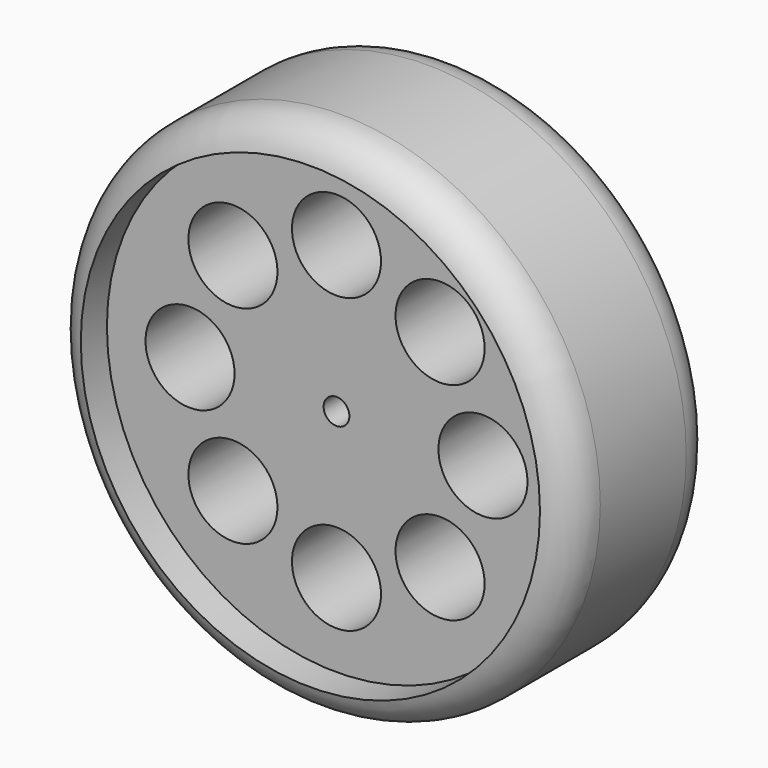
from build123d import *

# Parameters (mm, degrees)
F0_R     = 29.464
F0_R_2   = 5.715
F0_R_3   = 1.651
F1_DEPTH = 7.62
F0_R_4   = 33.274
F2_DEPTH = 11.811


# Not quite as in the source:
# - a fillet or chamfer that OpenCascade refuses, or shapes differently, is made with other operations: its cross-section is extruded or revolved along the edge and cut away or added


with BuildPart() as f1:
    # F0 (on Front) → F1 (new body, symmetric)
    with BuildSketch(Plane.XZ):
        Circle(F0_R)
        with Locations((-13.2907790592, -13.2907790592)):
            Circle(F0_R_2, mode=Mode.SUBTRACT)
        with Locations((0, -18.796)):
            Circle(F0_R_2, mode=Mode.SUBTRACT)
        with Locations((13.2907790592, -13.2907790592)):
            Circle(F0_R_2, mode=Mode.SUBTRACT)
        with Locations((-18.796, 0)):
            Circle(F0_R_2, mode=Mode.SUBTRACT)
        with Locations((-13.2907790592, 13.2907790592)):
            Circle(F0_R_2, mode=Mode.SUBTRACT)
        Circle(F0_R_3, mode=Mode.SUBTRACT)
        with Locations((13.2907790592, 13.2907790592)):
            Circle(F0_R_2, mode=Mode.SUBTRACT)
        with Locations((18.796, 0)):
            Circle(F0_R_2, mode=Mode.SUBTRACT)
        with Locations((0, 18.796)):
            Circle(F0_R_2, mode=Mode.SUBTRACT)
    extrude(amount=F1_DEPTH, both=True)

    # F0 (on Front) → F2 (join, symmetric)
    with BuildSketch(Plane.XZ):
        Circle(F0_R_4)
        Circle(F0_R, mode=Mode.SUBTRACT)
    extrude(amount=F2_DEPTH, both=True)

    # F3: fillet of radius 5.08 on 3 edges, made by hand

    # F3_s1 → F3_t2 (revolve, cut)
    with BuildSketch(Plane.XY):
        with BuildLine():
            ThreePointArc((33.274, 6.8923111503), (32.2100926284, 10.0031631237), (29.464, 11.811))
            Line((29.464, 11.811), (33.274, 11.811))
            Line((33.274, 11.811), (33.274, 6.8923111503))
        make_face()
    revolve(axis=Axis((0, 11.811, 0), (0, -1, 0)), mode=Mode.SUBTRACT)

    # F3_s3 → F3_t4 (revolve, cut)
    with BuildSketch(Plane.XY):
        with BuildLine():
            ThreePointArc((33.274, -6.8923111503), (32.2100926284, -10.0031631237), (29.464, -11.811))
            Line((29.464, -11.811), (33.274, -11.811))
            Line((33.274, -11.811), (33.274, -6.8923111503))
        make_face()
    revolve(axis=Axis((0, -11.811, 0), (0, -1, 0)), mode=Mode.SUBTRACT)


solid = f1.part
